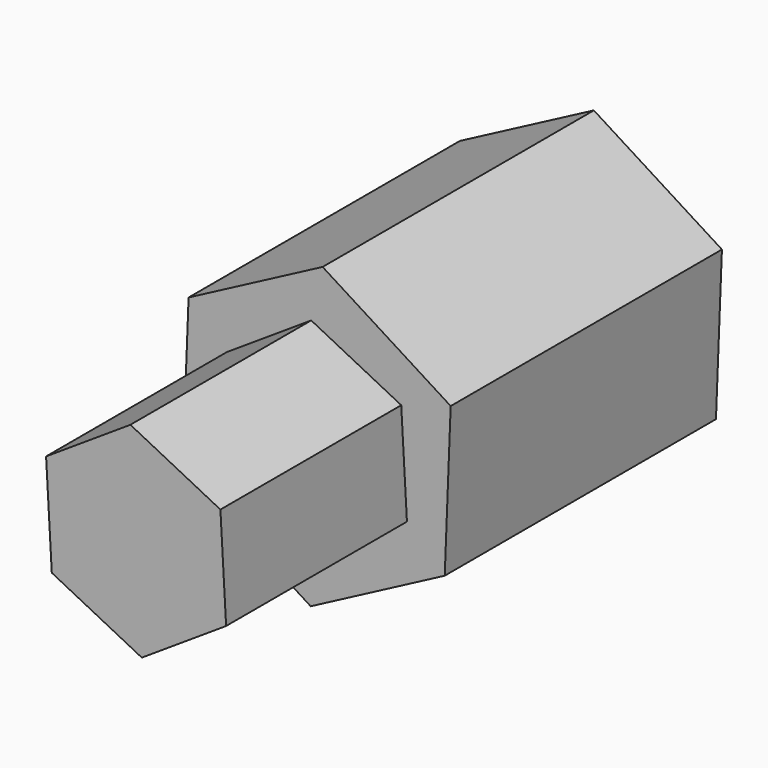
from build123d import *

# Parameters (mm, degrees)
F1_DEPTH = 15
F3_DEPTH = 10
F4_R     = 1.25
F5_DEPTH = 8


# Not quite as in the source:
# - ends of sketch curves that miss each other by under 0.0002 mm in the source are joined


with BuildPart() as f1:
    # F0 (on Front) → F1 (new body)
    with BuildSketch(Plane.XZ):
        Polygon((-5.7235665096, 3.5781680242), (-5.9874106989, -3.1166349037), (-0.3214230722, -6.6925111543), (5.608370415, -3.5735600573), (5.8721762755, 3.1212672902), (0.2061886488, 6.6971435408), align=None)
    extrude(amount=F1_DEPTH)

    # F2 (on face) → F3 (join)
    with BuildSketch(Plane.XZ.offset(15)):
        Polygon((-4.0286979474, 2.0048922286), (-3.7759230982, -2.4479388793), (0.2067050986, -4.4554086614), (3.9365390256, -2.0100863602), (3.6837447559, 2.442705723), (-0.2988834409, 4.4501755052), align=None)
    extrude(amount=F3_DEPTH)

    # F4 (on face) → F5 (cut)
    with BuildSketch(Plane(origin=(0, 0, 0), x_dir=(-1, 0, 0), z_dir=(0, 1, 0))):
        Circle(F4_R)
    extrude(amount=-F5_DEPTH, mode=Mode.SUBTRACT)


solid = f1.part
